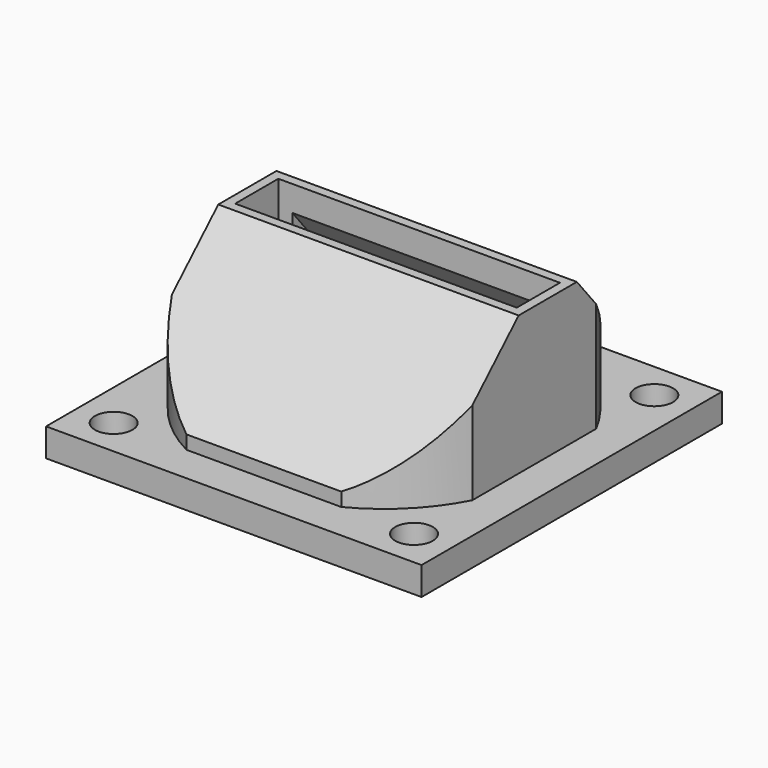
from build123d import *

# Parameters (mm, degrees)
F0_W          = 40
F0_H          = 40
F1_DEPTH      = 3
F2_R          = 2
F3_DEPTH      = 25
F5_DEPTH      = 30
F7_DEPTH      = 36.001
F9_DEPTH      = 36.001
F11_DEPTH     = 36.001
F12_T         = 2.5
F12_T3_DEPTH  = 21.4924225025
F12_T5_DEPTH  = 21.4924225025
F12_T8_ANGLE  = 35.4679110995
F12_T10_ANGLE = 35.4679110995
F12_T12_ANGLE = 35.4679110995
F12_T14_ANGLE = 35.4679110995
F13_W         = 30
F13_H         = 5.7462014769
F14_DEPTH     = 25


# Not quite as in the source:
# - a shell that OpenCascade refuses in one call is made with other operations: the cavity is built on its own and cut out


with BuildPart() as f1:
    # F0 (on Top) → F1 (new body)
    with BuildSketch(Plane.XY):
        with Locations((20, 20)):
            Rectangle(F0_W, F0_H)
    extrude(amount=F1_DEPTH)

    # F2 (on face) → F3 (cut)
    with BuildSketch(Plane.XY.offset(3)):
        with Locations((4, 36)):
            Circle(F2_R)
        with Locations((36, 36)):
            Circle(F2_R)
        with Locations((36, 4)):
            Circle(F2_R)
        with Locations((4, 4)):
            Circle(F2_R)
    extrude(amount=-F3_DEPTH, mode=Mode.SUBTRACT)

    # F4 (on face) → F5 (join)
    with BuildSketch(Plane.XY.offset(3)):
        with BuildLine():
            Line((28.2462112512, 36), (11.7537887488, 36))
            ThreePointArc((11.7537887488, 36), (7.2720779386, 32.7279220614), (4, 28.2462112512))
            Line((4, 28.2462112512), (4, 11.7537887488))
            ThreePointArc((4, 11.7537887488), (7.2720779386, 7.2720779386), (11.7537887488, 4))
            Line((11.7537887488, 4), (28.2462112512, 4))
            ThreePointArc((28.2462112512, 4), (32.7279220614, 7.2720779386), (36, 11.7537887488))
            Line((36, 11.7537887488), (36, 28.2462112512))
            ThreePointArc((36, 28.2462112512), (32.7279220614, 32.7279220614), (28.2462112512, 36))
        make_face()
    extrude(amount=F5_DEPTH)

    # F6 (on face) → F7 (cut, through all)
    with BuildSketch(Plane.YZ.offset(36)):
        Polygon((2.4936108384, 3), (39.5666994154, 38.5907627642), (48.4694316983, 41.8781600893), (2.4936108384, 41.8781600893), align=None)
    extrude(amount=-F7_DEPTH, mode=Mode.SUBTRACT)

    # F8 (on face) → F9 (cut, through all)
    with BuildSketch(Plane.YZ.offset(36)):
        Polygon((20.7161400467, 23.8601379097), (36.8017591536, 4.2844121344), (40.8149436116, 38.1976142526), (20.7161400467, 38.1976142526), align=None)
    extrude(amount=-F9_DEPTH, mode=Mode.SUBTRACT)

    # F10 (on face) → F11 (cut, through all)
    with BuildSketch(Plane.YZ.offset(36)):
        Polygon((13.3647378534, 17.821257934), (36.5101168772, 17.821257934), (38.6116616428, 31.5769352019), (13.3647378534, 31.5769352019), align=None)
    extrude(amount=-F11_DEPTH, mode=Mode.SUBTRACT)

    # F12: shell of thickness 2.5, made by hand


with BuildPart() as f12_core1:
    # F12_t2: copy of F1
    add(f1.part)

    # the walls: a layer under each face that stays
    f12_faces = [f12_core1.faces().sort_by_distance(p)[0] for p in [
        (0, 20, 1.5),
        (20, 40, 1.5),
        (20, 0, 1.5),
        (6.6666666667, 6.6666666667, 3),
        (40, 20, 1.5),
        (2, 4, 1.5),
        (34, 4, 1.5),
        (2, 36, 1.5),
        (34, 36, 1.5),
        (36, 20, 10.410628967),
        (32.7279220614, 7.2720779386, 7.444960048),
        (32.7279220614, 32.7279220614, 8.8481312629),
        (20, 4, 3.7230789413),
        (20, 36, 4.1300647323),
        (7.2720779386, 7.2720779386, 7.444960048),
        (7.2720779386, 32.7279220614, 8.8481312629),
        (4, 20, 10.410628967),
        (20, 30.8391816878, 11.5406936993),
        (20, 21.8052626371, 17.821257934),
        (20, 10.9660809493, 11.1337079083),
    ]]
    thicken(f12_faces, amount=-F12_T, mode=Mode.SUBTRACT)

    # F12_s4 → F12_t3 (cut)
    with BuildSketch(Plane.XZ.offset(-30.7462112512)):
        Polygon((36.025, 3.025), (36, 0.5), (33.5, 0.5), (33.5, 3), align=None)
        Polygon((3.975, 3.025), (4, 0.5), (6.5, 0.5), (6.5, 3), align=None)
    extrude(amount=F12_T3_DEPTH, mode=Mode.SUBTRACT)

    # F12_s6 → F12_t5 (cut)
    with BuildSketch(Plane.YZ.offset(9.2537887488)):
        Polygon((3.975, 3.025), (4, 0.5), (6.5, 0.5), (6.5, 3), align=None)
        Polygon((36.025, 3.025), (36, 0.5), (33.5, 0.5), (33.5, 3), align=None)
    extrude(amount=F12_T5_DEPTH, mode=Mode.SUBTRACT)

    # F12_s7 → F12_t8 (revolve, cut)
    with BuildSketch(Plane(origin=(23.9468753099, 12.3419370383, 0), x_dir=(0, 0, 1), z_dir=(-0.8888888889, -0.4581228473, 0))):
        Polygon((3.025, -9.409679168), (0.5, -9.384679168), (0.5, -6.884679168), (3, -6.884679168), align=None)
    revolve(axis=Axis((20, 20, 3), (0, 0, 1)), revolution_arc=F12_T8_ANGLE, mode=Mode.SUBTRACT)

    # F12_s9 → F12_t10 (revolve, cut)
    with BuildSketch(Plane(origin=(-3.9468753099, 7.6580629617, 0), x_dir=(0, 0, 1), z_dir=(0.4581228473, -0.8888888889, 0))):
        Polygon((3.025, -44.9652347236), (0.5, -44.9402347236), (0.5, -42.4402347236), (3, -42.4402347236), align=None)
    revolve(axis=Axis((20, 20, 3), (0, 0, 1)), revolution_arc=F12_T10_ANGLE, mode=Mode.SUBTRACT)

    # F12_s11 → F12_t12 (revolve, cut)
    with BuildSketch(Plane(origin=(-3.9468753099, 7.6580629617, 0), x_dir=(0, 0, 1), z_dir=(-0.4581228473, 0.8888888889, 0))):
        Polygon((3.025, 8.9152347236), (0.5, 8.9402347236), (0.5, 11.4402347236), (3, 11.4402347236), align=None)
    revolve(axis=Axis((20, 20, 3), (0, 0, 1)), revolution_arc=F12_T12_ANGLE, mode=Mode.SUBTRACT)

    # F12_s13 → F12_t14 (revolve, cut)
    with BuildSketch(Plane(origin=(23.9468753099, 12.3419370383, 0), x_dir=(0, 0, 1), z_dir=(0.8888888889, 0.4581228473, 0))):
        Polygon((3.025, -26.640320832), (0.5, -26.615320832), (0.5, -24.115320832), (3, -24.115320832), align=None)
    revolve(axis=Axis((20, 20, 3), (0, 0, 1)), revolution_arc=F12_T14_ANGLE, mode=Mode.SUBTRACT)


with BuildPart() as f1_1:
    add(f1.part)

    # what is left inside the walls is the cavity
    f12_cavity = [f12_core1.part.solids().sort_by_distance(p)[0] for p in [
        (20, 14.166667, 0.025),
    ]]
    add(f12_cavity, mode=Mode.SUBTRACT)

    # F13 (on face) → F14 (cut)
    with BuildSketch(Plane.XY.offset(17.821257934)):
        with Locations((20, 21.8052626371)):
            Rectangle(F13_W, F13_H)
    extrude(amount=-F14_DEPTH, mode=Mode.SUBTRACT)


solid = f1_1.part
